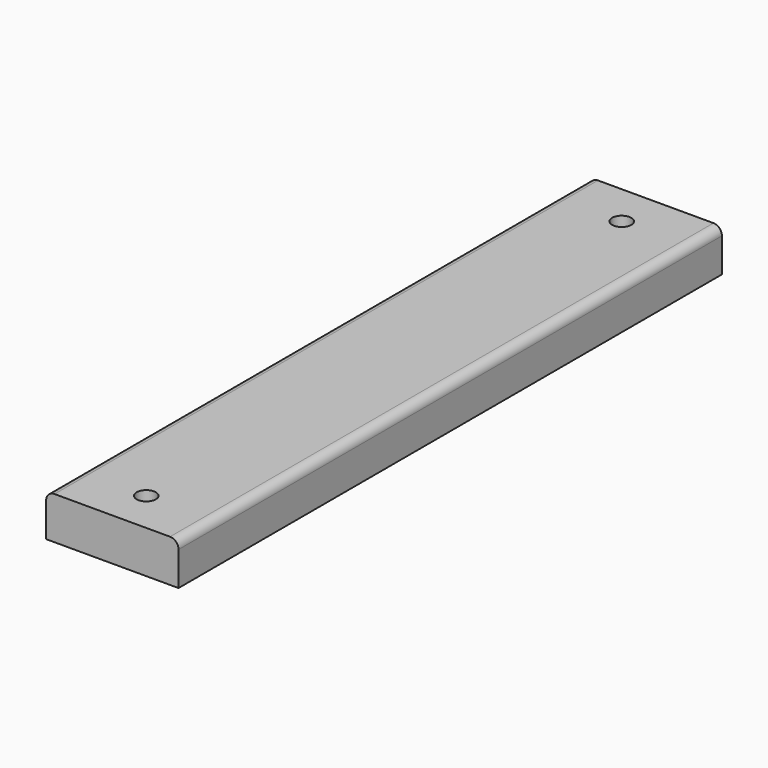
from build123d import *

# Parameters (mm, degrees)
F0_W     = 15.6
F0_H     = 5
F1_DEPTH = 40
F2_R     = 1
F3_R     = 1
F8_D     = 2.2606
F10_D    = 2.2606


# Not quite as in the source:
# - a feature of the source that left no trace in its solid (it failed there, or was rolled back) is left out


with BuildPart() as f1:
    # F0 (on Front) → F1 (new body, symmetric)
    with BuildSketch(Plane.XZ):
        with Locations((0, 5.57)):
            Rectangle(F0_W, F0_H)
    extrude(amount=F1_DEPTH, both=True)

    # F2
    f2_edges = [f1.edges().sort_by_distance(p)[0] for p in [
        (7.8, 0, 8.07),
    ]]
    fillet(f2_edges, radius=F2_R)

    # F3
    f3_edges = [f1.edges().sort_by_distance(p)[0] for p in [
        (-7.8, 0, 8.07),
    ]]
    fillet(f3_edges, radius=F3_R)

    # F8 (through all)
    with Locations(Plane(origin=(0, 0, 0), x_dir=(1, 0, 0), z_dir=(0, 0, -1))):
        with Locations((0, 35)):
            Hole(F8_D / 2)

    # F10 (through all)
    with Locations(Plane(origin=(0, 0, 0), x_dir=(1, 0, 0), z_dir=(0, 0, -1))):
        with Locations((0, -35)):
            Hole(F10_D / 2)


solid = f1.part
